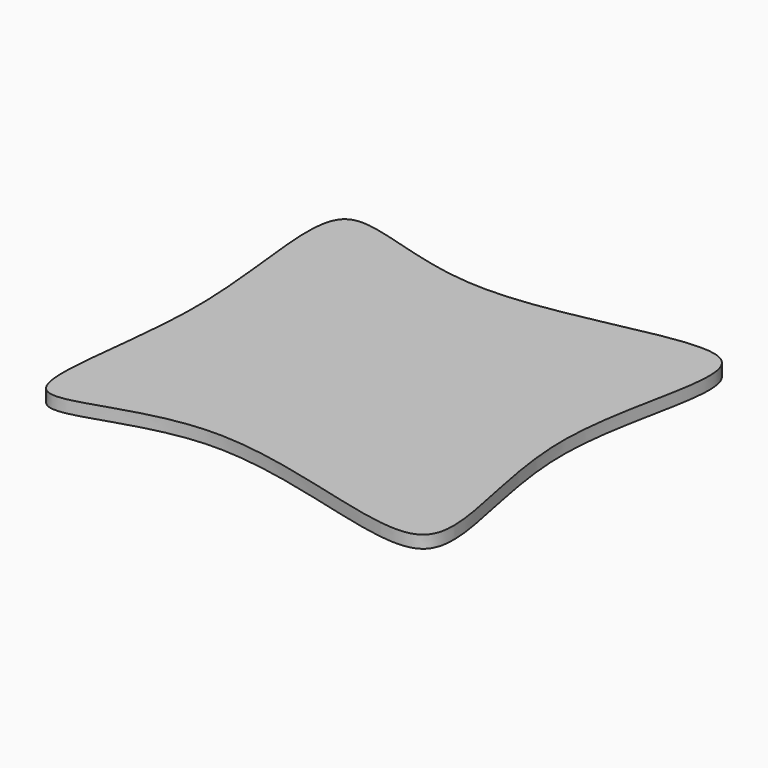
from build123d import *

# Parameters (mm, degrees)
F1_DEPTH = 5


with BuildPart() as f1:
    # F0 (on Top) → F1 (new body)
    with BuildSketch(Plane.XY):
        with BuildLine():
            add(Edge.make_bspline(
                [(-76.1707425117, 75.3596574068), (-67.9968433933, 82.069460697), (-15.597524702, 48.6398863375), (103.5217379606, 101.6867901375), (55.216921862, 0.2881885102), (105.9306861891, -106.7784298577), (-18.988575814, -44.0566610203), (-93.5708466547, -96.7549538222), (-65.6195621806, 0.3174841959), (-85.2030712458, 67.9451850503), (-76.1707425117, 75.3596574068)],
                knots=[0, 0, 0, 0, 0.1129783204, 0.2504267288, 0.3746317241, 0.5005723819, 0.6416864135, 0.7518498038, 0.8751566033, 1, 1, 1, 1], degree=3))
        make_face()
    extrude(amount=F1_DEPTH)


solid = f1.part
